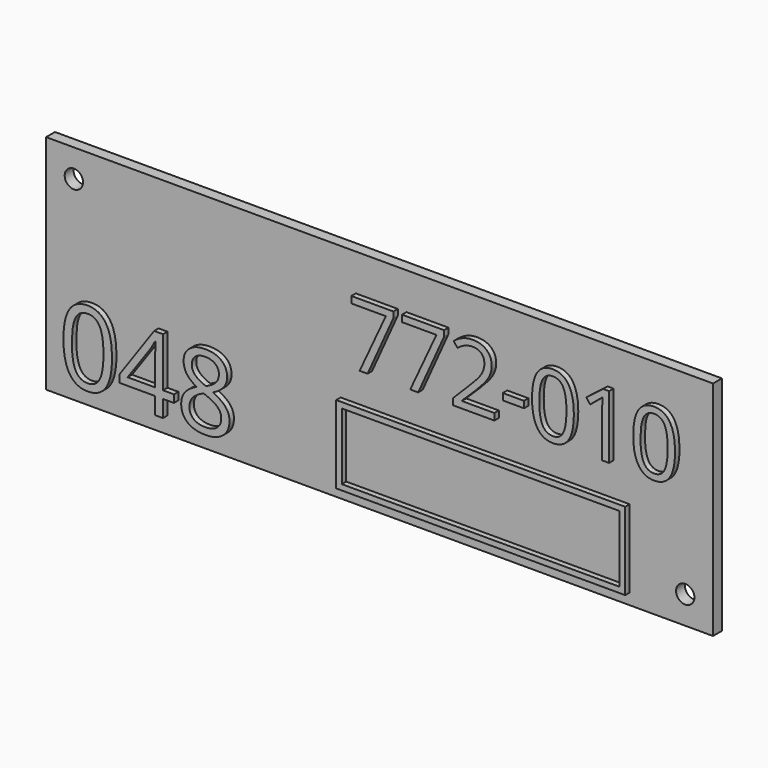
from build123d import *

# Parameters (mm, degrees)
F0_W         = 120
F0_H         = 40
F1_DEPTH     = 2
F3_D         = 3.3
F4_TEXT_SIZE = 15.9270012443
F5_DEPTH     = 1
F6_TEXT_SIZE = 18.5155049272
F7_DEPTH     = 1
F8_W         = 52
F8_H         = 14
F8_W_2       = 49.99999962
F8_H_2       = 11.99999962
F9_DEPTH     = 1


# Not quite as in the source:
# - Text() gives the source's letters only with a copy of the font that has no kerning and outlines rounded to 1/6400 em; it was checked with that copy


with BuildPart() as f1:
    # F0 (on Front) → F1 (new body)
    with BuildSketch(Plane.XZ):
        Rectangle(F0_W, F0_H)
    extrude(amount=F1_DEPTH)

    # F3 (through all)
    with Locations(Plane.XZ.offset(2)):
        with Locations((-55, 15), (55, -15)):
            Hole(F3_D / 2)

    # F4 (on face) → F5 (join)
    with BuildSketch(Plane.XZ.offset(2)):
        with Locations((-5, 2)):
            Text('772-010', F4_TEXT_SIZE, font='Open Sans', text_align=(TextAlign.LEFT, TextAlign.BOTTOM))
    extrude(amount=F5_DEPTH)

    # F6 (on face) → F7 (join)
    with BuildSketch(Plane.XZ.offset(2)):
        with Locations((-57, -17)):
            Text('048', F6_TEXT_SIZE, font='Open Sans', text_align=(TextAlign.LEFT, TextAlign.BOTTOM))
    extrude(amount=F7_DEPTH)

    # F8 (on face) → F9 (join)
    with BuildSketch(Plane.XZ.offset(2)):
        with Locations((19, -11)):
            Rectangle(F8_W, F8_H)
        with Locations((19, -11)):
            Rectangle(F8_W_2, F8_H_2, mode=Mode.SUBTRACT)
    extrude(amount=F9_DEPTH)


solid = f1.part
